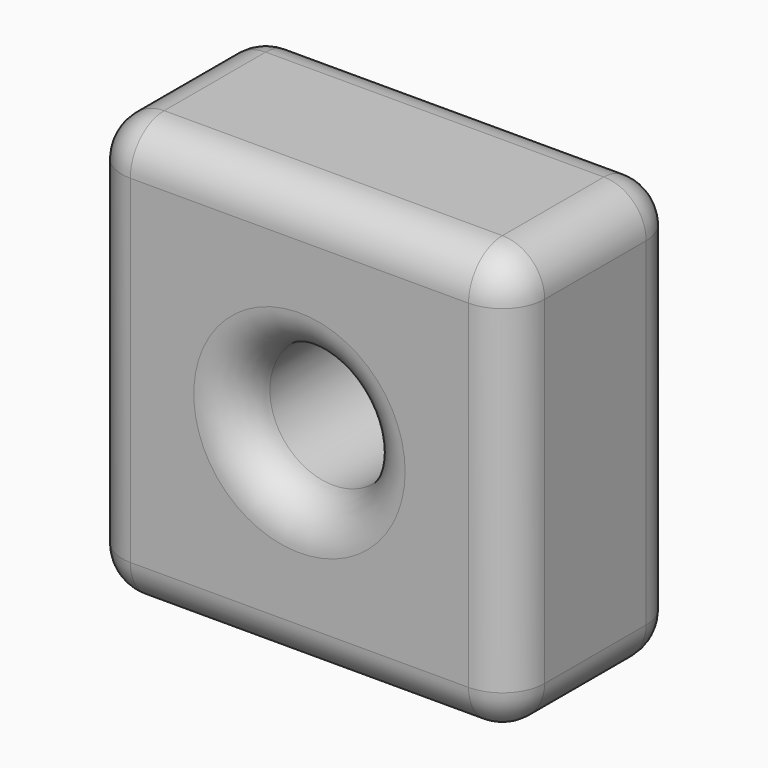
from build123d import *

# Parameters (mm, degrees)
F0_W     = 100
F0_H     = 100
F0_R     = 15
F1_DEPTH = 50
F2_R     = 10
F3_DEPTH = 50
F6_R     = 10


# Not quite as in the source:
# - the program builds the solid bodies; features that only make, move or delete a surface that nothing else refers to are left out


with BuildPart() as f1:
    # F0 (on Front) → F1 (new body, symmetric)
    with BuildSketch(Plane.XZ):
        Rectangle(F0_W, F0_H)
        Circle(F0_R, mode=Mode.SUBTRACT)
    extrude(amount=F1_DEPTH, both=True)

    # F2
    f2_edges = [f1.edges().sort_by_distance(p)[0] for p in [
        (50, 50, 0),
        (50, 0, 50),
        (50, -50, 0),
        (50, 0, -50),
        (0, -50, 50),
        (-50, -50, 0),
        (0, -50, -50),
        (-15, -50, 0),
        (0, 50, 50),
        (-50, 0, 50),
        (-50, 50, 0),
        (-50, 0, -50),
    ]]
    fillet(f2_edges, radius=F2_R)

    # F0 (on Front) → F3 (cut)
    with BuildSketch(Plane.XZ):
        Rectangle(F0_W, F0_H)
        Circle(F0_R, mode=Mode.SUBTRACT)
    extrude(amount=-F3_DEPTH, mode=Mode.SUBTRACT)

    # F6
    f6_edges = [f1.edges().sort_by_distance(p)[0] for p in [
        (-47.071068, 0, -47.071068),
        (-40, -20, -50),
        (-47.071068, -40, -47.071068),
        (-50, -20, -40),
        (-47.071068, 0, 47.071068),
        (-40, -20, 50),
        (-47.071068, -40, 47.071068),
        (-50, -20, 40),
        (-47.071068, -47.071068, 40),
        (-50, -40, 0),
        (-40, -50, 0),
        (-47.071068, -47.071068, -40),
        (-50, 0, 0),
        (47.071068, -40, -47.071068),
        (50, -20, -40),
        (47.071068, 0, -47.071068),
        (40, -20, -50),
        (50, -40, 0),
        (50, -20, 40),
        (50, 0, 0),
        (40, -50, 0),
        (0, -50, -40),
        (0, -50, 40),
        (-25, -50, 0),
        (0, 0, 50),
        (47.071068, 0, 47.071068),
        (0, 0, -50),
    ]]
    fillet(f6_edges, radius=F6_R)


solid = f1.part
